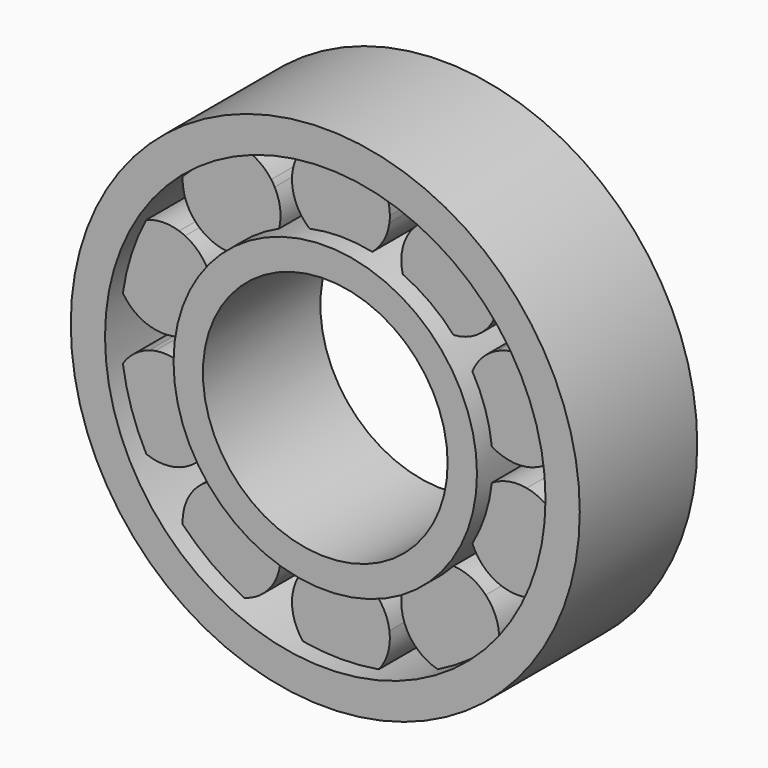
from build123d import *

# Parameters (mm, degrees)
F0_R     = 26
F0_R_2   = 22.5
F1_DEPTH = 15
F0_R_3   = 15.5
F0_R_4   = 12.5
F4_DEPTH = 5.5
F5_COUNT = 10


with BuildPart() as f1:
    # F0 (on Front) → F1 (new body)
    with BuildSketch(Plane.XZ):
        Circle(F0_R)
        Circle(F0_R_2, mode=Mode.SUBTRACT)
    extrude(amount=F1_DEPTH)



with BuildPart() as f1b:
    # F0 (on Front) → F1, piece 2 (new body)
    with BuildSketch(Plane.XZ):
        Circle(F0_R_3)
        Circle(F0_R_4, mode=Mode.SUBTRACT)
    extrude(amount=F1_DEPTH)


with BuildPart() as f1_1:
    add(f1.part)

    add(f1b.part)  # F4 merges F1b
    # F3 (on offset) → F4 (join, symmetric)
    with BuildSketch(Plane.XZ.offset(7.5)):
        with BuildLine():
            ThreePointArc((-4.956528, 18.342105), (0, 19), (4.956528, 18.342105))
            ThreePointArc((4.956528, 18.342105), (4.98912, 18.670335), (5, 19))
            ThreePointArc((5, 19), (-0.329665, 23.98912), (-4.956528, 18.342105))
        make_face()
        with BuildLine():
            ThreePointArc((-4.956528, 18.342105), (0, 14), (4.956528, 18.342105))
            ThreePointArc((4.956528, 18.342105), (0, 19), (-4.956528, 18.342105))
        make_face()
    extrude(amount=F4_DEPTH, both=True)

    # F5: F1 ×10 about axis
    f5_axis = Axis((0, -15, 0), (0, -1, 0))


with BuildPart() as f1_2:
    add(f1_1.part)
    for i in range(1, F5_COUNT):
        add(f1_1.part.rotate(f5_axis, i * 360 / F5_COUNT))


solid = f1_2.part
